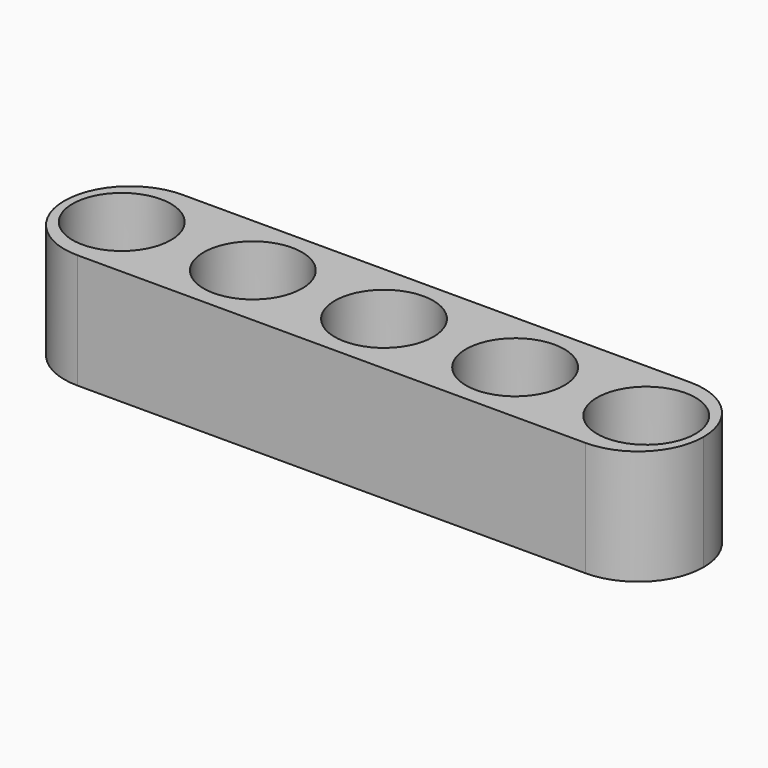
from build123d import *

# Parameters (mm, degrees)
F0_W     = 39
F0_H     = 8
F0_R     = 3
F1_DEPTH = 7
F2_R     = 3.99999


# Not quite as in the source:
# - a fillet or chamfer is up to 0.001 mm smaller than in the source, because OpenCascade refuses the exact size


with BuildPart() as f1:
    # F0 (on Top) → F1 (new body)
    with BuildSketch(Plane.XY):
        Rectangle(F0_W, F0_H)
        with Locations((-16, 0)):
            Circle(F0_R, mode=Mode.SUBTRACT)
        with Locations((-8, 0)):
            Circle(F0_R, mode=Mode.SUBTRACT)
        Circle(F0_R, mode=Mode.SUBTRACT)
        with Locations((8, 0)):
            Circle(F0_R, mode=Mode.SUBTRACT)
        with Locations((16, 0)):
            Circle(F0_R, mode=Mode.SUBTRACT)
    extrude(amount=F1_DEPTH)

    # F2 (radius 4 in the source; OpenCascade refuses exactly that, so slightly less here)
    f2_edges = [f1.edges().sort_by_distance(p)[0] for p in [
        (-19.5, 4, 3.5),
        (-19.5, -4, 3.5),
        (19.5, -4, 3.5),
        (19.5, 4, 3.5),
    ]]
    fillet(f2_edges, radius=F2_R)


solid = f1.part
